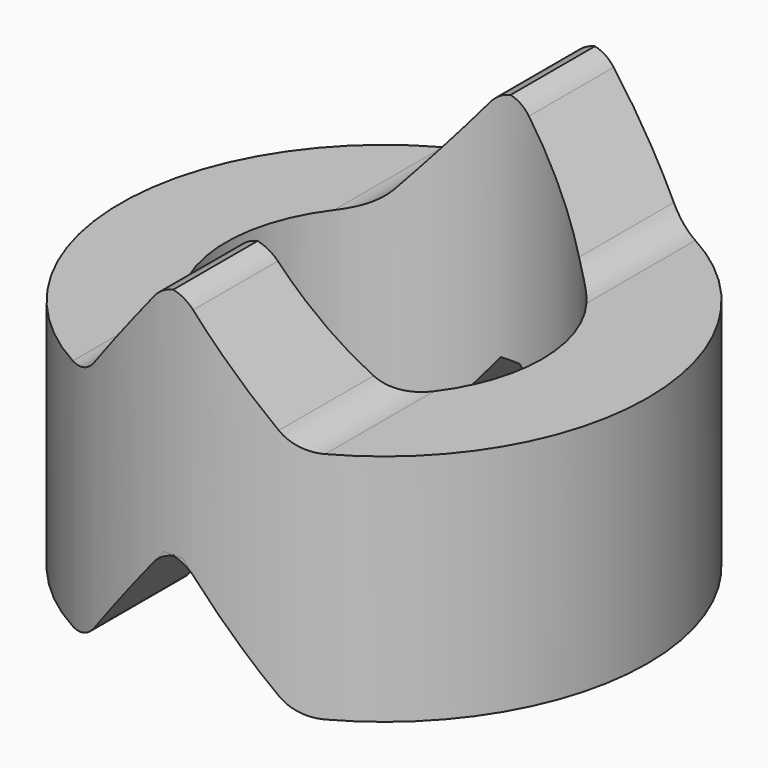
from build123d import *

# Parameters (mm, degrees)
F0_R         = 38.1
F0_R_2       = 22.86
F1_DEPTH     = 127
F4_DEPTH     = 80.011
F5_T4_DEPTH  = 27.2677982704
F5_S5_R      = 38.1
F5_T6_DEPTH  = 15
F5_S7_R      = 22.86
F5_T8_DEPTH  = 15
F5_T12_DEPTH = 27.2677982704
F5_S13_R     = 38.1
F5_T14_DEPTH = 15
F5_S15_R     = 22.86
F5_T16_DEPTH = 15
F5_T17_DEPTH = 27.2653813946
F5_T19_DEPTH = 27.2653813946


# Not quite as in the source:
# - a fillet or chamfer that OpenCascade refuses, or shapes differently, is made with other operations: its cross-section is extruded or revolved along the edge and cut away or added


with BuildPart() as f1:
    # F0 (on Top) → F1 (new body)
    with BuildSketch(Plane.XY):
        Circle(F0_R)
        Circle(F0_R_2, mode=Mode.SUBTRACT)
    extrude(amount=F1_DEPTH)

    # F3 (on offset) → F4 (cut, through all)
    with BuildSketch(Plane.XZ.offset(41.91)):
        with BuildLine():
            Line((1.3741332924, 44.0691516455), (0, 44.0691516455))
            Line((0, 44.0691516455), (0, 27.1781024958))
            Line((0, 27.1781024958), (0, -6.6039958037))
            Line((0, -6.6039958037), (38.1, -6.6039958037))
            Line((38.1, -6.6039958037), (38.1, 27.1781024958))
            Line((38.1, 27.1781024958), (18.242812226, 27.1781024958))
            ThreePointArc((18.242812226, 27.1781024958), (15.5282171859, 27.7875908663), (13.3347289514, 29.4990556395))
            Line((13.3347289514, 29.4990556395), (1.3741332924, 44.0691516455))
        make_face()
        with BuildLine():
            Line((0, 44.0691516455), (-1.3741332924, 44.0691516455))
            Line((-1.3741332924, 44.0691516455), (-13.3347289514, 29.4990556395))
            ThreePointArc((-13.3347289514, 29.4990556395), (-15.5282171859, 27.7875908663), (-18.242812226, 27.1781024958))
            Line((-18.242812226, 27.1781024958), (-38.1, 27.1781024958))
            Line((-38.1, 27.1781024958), (-38.1, -6.6039958037))
            Line((-38.1, -6.6039958037), (0, -6.6039958037))
            Line((0, -6.6039958037), (0, 27.1781024958))
            Line((0, 27.1781024958), (0, 44.0691516455))
        make_face()
        with BuildLine():
            Line((38.1, 60.9602007953), (38.1, 77.9781024958))
            Line((38.1, 77.9781024958), (1.27, 77.9781024958))
            Line((1.27, 77.9781024958), (1.2895432809, 77.9542953638))
            Line((1.2895432809, 77.9542953638), (13.3347289514, 63.281153939))
            ThreePointArc((13.3347289514, 63.281153939), (15.5282171859, 61.5696891658), (18.242812226, 60.9602007953))
            Line((18.242812226, 60.9602007953), (38.1, 60.9602007953))
        make_face()
        with BuildLine():
            Line((-38.1, 77.9781024958), (-38.1, 60.9602007953))
            Line((-38.1, 60.9602007953), (-18.242812226, 60.9602007953))
            ThreePointArc((-18.242812226, 60.9602007953), (-15.5282171859, 61.5696891658), (-13.3347289514, 63.281153939))
            Line((-13.3347289514, 63.281153939), (-1.2895432809, 77.9542953638))
            Line((-1.2895432809, 77.9542953638), (-1.27, 77.9781024958))
            Line((-1.27, 77.9781024958), (-38.1, 77.9781024958))
        make_face()
        Polygon((-38.1, 131.2988996506), (-38.1, 77.9781024958), (-1.27, 77.9781024958), (-1.2391987117, 77.9781024958), (-0.1262114529, 77.9781024958), (0, 77.9781024958), (1.2391987117, 77.9781024958), (1.27, 77.9781024958), (38.1, 77.9781024958), (38.1, 80.6030047561), (38.1, 131.2988996506), align=None)
    extrude(amount=-F4_DEPTH, mode=Mode.SUBTRACT)

    # F5: fillet of radius 5.08 on 6 edges, made by hand


with BuildPart() as f5_tool2:
    # F5_s3 → F5_t4 (new body)
    with BuildSketch(Plane.XZ.offset(44.0808363055)):
        with BuildLine():
            ThreePointArc((-1.0281164884, 44.0691516455), (1.1435595437, 43.5815609491), (2.8983501313, 42.2123891305))
            Line((2.8983501313, 42.2123891305), (1.3741332924, 44.0691516455))
            Line((1.3741332924, 44.0691516455), (-1.0281164884, 44.0691516455))
        make_face()
    extrude(amount=-F5_T4_DEPTH)

    # F5_s5 → F5_t6 (intersect, symmetric)
    with BuildSketch(Plane.XY.offset(43.1)):
        Circle(F5_S5_R)
    extrude(amount=F5_T6_DEPTH, both=True, mode=Mode.INTERSECT)

    # F5_s7 → F5_t8 (cut, symmetric)
    with BuildSketch(Plane.XY.offset(43.1)):
        Circle(F5_S7_R)
    extrude(amount=F5_T8_DEPTH, both=True, mode=Mode.SUBTRACT)


with BuildPart() as f1_1:
    add(f1.part)

    # F5_t1: union F5_tool2
    add(f5_tool2.part)


with BuildPart() as f5_tool10:
    # F5_s11 → F5_t12 (new body)
    with BuildSketch(Plane.XZ.offset(44.0808363055)):
        with BuildLine():
            ThreePointArc((-2.8983501313, 42.2123891305), (-1.1435595437, 43.5815609491), (1.0281164884, 44.0691516455))
            Line((1.0281164884, 44.0691516455), (-1.3741332924, 44.0691516455))
            Line((-1.3741332924, 44.0691516455), (-2.8983501313, 42.2123891305))
        make_face()
    extrude(amount=-F5_T12_DEPTH)

    # F5_s13 → F5_t14 (intersect, symmetric)
    with BuildSketch(Plane.XY.offset(43.1)):
        Circle(F5_S13_R)
    extrude(amount=F5_T14_DEPTH, both=True, mode=Mode.INTERSECT)

    # F5_s15 → F5_t16 (cut, symmetric)
    with BuildSketch(Plane.XY.offset(43.1)):
        Circle(F5_S15_R)
    extrude(amount=F5_T16_DEPTH, both=True, mode=Mode.SUBTRACT)


with BuildPart() as f1_2:
    add(f1_1.part)

    # F5_t9: union F5_tool10
    add(f5_tool10.part)

    # F5_s18 → F5_t17 (cut)
    with BuildSketch(Plane.XZ.offset(16.8190705077)):
        with BuildLine():
            ThreePointArc((2.7942168389, 76.1213399807), (1.0394262513, 77.4905117994), (-1.1322497808, 77.9781024958))
            Line((-1.1322497808, 77.9781024958), (1.27, 77.9781024958))
            Line((1.27, 77.9781024958), (2.7942168389, 76.1213399807))
        make_face()
        with BuildLine():
            ThreePointArc((1.1322497808, 77.9781024958), (-1.0394262513, 77.4905117994), (-2.7942168389, 76.1213399807))
            Line((-2.7942168389, 76.1213399807), (-1.27, 77.9781024958))
            Line((-1.27, 77.9781024958), (1.1322497808, 77.9781024958))
        make_face()
    extrude(amount=F5_T17_DEPTH, mode=Mode.SUBTRACT)

    # F5_s20 → F5_t19 (cut)
    with BuildSketch(Plane.XZ.offset(-44.0844519023)):
        with BuildLine():
            ThreePointArc((-1.1322497808, 77.9781024958), (1.0394262513, 77.4905117994), (2.7942168389, 76.1213399807))
            Line((2.7942168389, 76.1213399807), (1.27, 77.9781024958))
            Line((1.27, 77.9781024958), (-1.1322497808, 77.9781024958))
        make_face()
        with BuildLine():
            ThreePointArc((-2.7942168389, 76.1213399807), (-1.0394262513, 77.4905117994), (1.1322497808, 77.9781024958))
            Line((1.1322497808, 77.9781024958), (-1.27, 77.9781024958))
            Line((-1.27, 77.9781024958), (-2.7942168389, 76.1213399807))
        make_face()
    extrude(amount=F5_T19_DEPTH, mode=Mode.SUBTRACT)


solid = f1_2.part
